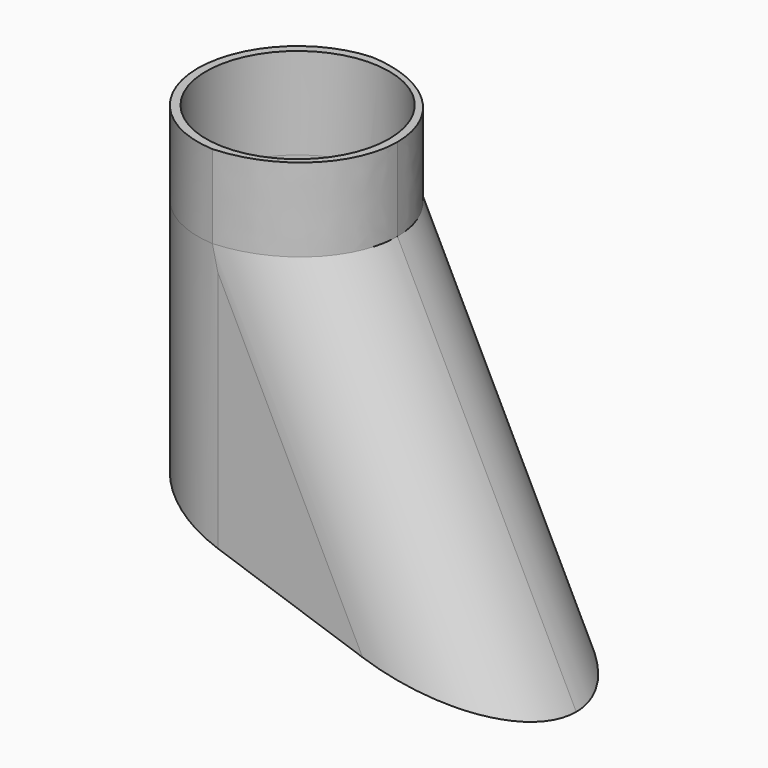
from build123d import *
from build123d import SkipClean  # not in build123d's __all__

# Parameters (mm, degrees)
F1_DEPTH    = 76.2
F2_T1_DEPTH = 279.4
F2_T3_DEPTH = 344.0535746512
F3_T        = -3.175
F5_DEPTH    = 31.75
F6_R        = 34.925
F7_DEPTH    = 38.1


# Not quite as in the source:
# - a fillet or chamfer that OpenCascade refuses, or shapes differently, is made with other operations: its cross-section is extruded or revolved along the edge and cut away or added


with BuildPart() as f1:
    # F0 (on Front) → F1 (new body)
    with BuildSketch(Plane.XZ):
        Polygon((144.4205327875, -48.6669262372), (76.2, 88.9), (0, 88.9), (0, 0), align=None)
    extrude(amount=-F1_DEPTH)

    # F2: fillet of radius 38.1 on 4 edges, made by hand

    # F2_s2 → F2_t1 (cut)
    with BuildSketch(Plane.XY.offset(-95.25)):
        with BuildLine():
            ThreePointArc((0, 38.1), (11.1592316368, 11.1592316368), (38.1, 0))
            Line((38.1, 0), (0, 0))
            Line((0, 0), (0, 38.1))
        make_face()
        with BuildLine():
            ThreePointArc((0, 38.1), (11.1592316368, 65.0407683632), (38.1, 76.2))
            Line((38.1, 76.2), (0, 76.2))
            Line((0, 76.2), (0, 38.1))
        make_face()
    extrude(amount=F2_T1_DEPTH, mode=Mode.SUBTRACT)

    # F2_s4 → F2_t3 (cut)
    with BuildSketch(Plane(origin=(90.1943185968, 0, -181.8771367864), x_dir=(0, 1, 0), z_dir=(-0.4442783761, 0, 0.8958887903))):
        with BuildLine():
            ThreePointArc((38.1, -107.7630734528), (65.0407683632, -96.603841816), (76.2, -69.6630734528))
            Line((76.2, -69.6630734528), (76.2, -107.7630734528))
            Line((76.2, -107.7630734528), (38.1, -107.7630734528))
        make_face()
        with BuildLine():
            ThreePointArc((38.1, -107.7630734528), (11.1592316368, -96.603841816), (0, -69.6630734528))
            Line((0, -69.6630734528), (0, -107.7630734528))
            Line((0, -107.7630734528), (38.1, -107.7630734528))
        make_face()
    extrude(amount=F2_T3_DEPTH, mode=Mode.SUBTRACT)

    # F3
    f3_openings = [f1.faces().sort_by_distance(p)[0] for p in [
        (71.049342, 38.1, -23.942254),
    ]]
    offset(amount=F3_T, openings=f3_openings)

    # F4 (on face) → F5 (join)
    with BuildSketch(Plane.XY.offset(88.9)):
        with BuildLine():
            add(Edge.make_bspline(
                [(36.0077691103, 0.0574899631), (76.1999999999, 2.0378158336), (76.2, 38.1)],
                knots=[4.7673308141, 4.7673308141, 4.7673308141, 6.2831853072, 6.2831853072, 6.2831853072], degree=2, weights=[1, 0.726262417, 1]))
            add(Edge.make_bspline(
                [(76.2, 38.1), (76.1999999999, 74.1621841664), (36.0077691103, 76.1425100369)],
                knots=[0, 0, 0, 1.5158544931, 1.5158544931, 1.5158544931], degree=2, weights=[1, 0.726262417, 1]))
            ThreePointArc((36.0077691103, 76.1425100369), (10.4294019138, 64.2906090336), (0, 38.1))
            ThreePointArc((0, 38.1), (10.4294019138, 11.9093909664), (36.0077691103, 0.0574899631))
        make_face()
    extrude(amount=F5_DEPTH)

    # F6 (on face) → F7 (cut)
    with BuildSketch(Plane.XY.offset(120.65)):
        with Locations((38.1, 38.1)):
            Circle(F6_R)
    with SkipClean():  # cleaning this boolean's faces spoils the solid; the shape is the same uncleaned
        extrude(amount=-F7_DEPTH, mode=Mode.SUBTRACT)


solid = f1.part
